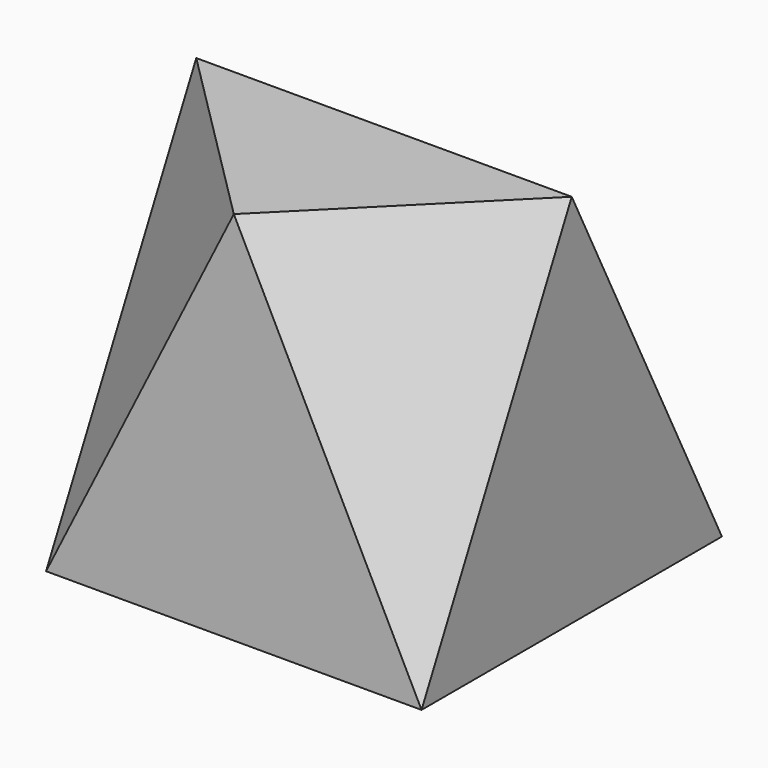
from build123d import *

# Parameters (mm, degrees)
F1_DEPTH = 20
F5_DEPTH = 13.3343333333


# Not quite as in the source:
# - a pattern or mirror of a feature is missing from the dataset's text; its kind, count and spacing are read off the source's solid


with BuildPart() as f1:
    # F0 (on Right) → F1 (new body, symmetric)
    with BuildSketch(Plane.YZ):
        Polygon((0, 40), (0, 0), (40, 0), (20, 40), align=None)
    extrude(amount=F1_DEPTH, both=True)

    # F4 (on 3pt) → F5 (cut, through all)
    with BuildSketch(Plane(origin=(8.8888888889, -8.8888888889, 4.4444444444), x_dir=(-0.7453559925, -0.596284794, 0.298142397), z_dir=(-0.6666666667, 0.6666666667, -0.3333333333))):
        Polygon((-14.90711985, 0), (11.92569588, 35.77708764), (-14.90711985, 44.72135955), align=None)
    f5 = extrude(amount=-F5_DEPTH, mode=Mode.SUBTRACT)

    # F5_copies: F5 across plane
    add(f5.mirror(Plane(origin=(0, 0, 0), x_dir=(0, 0, -1), z_dir=(-1, 0, 0))), mode=Mode.SUBTRACT)


solid = f1.part
